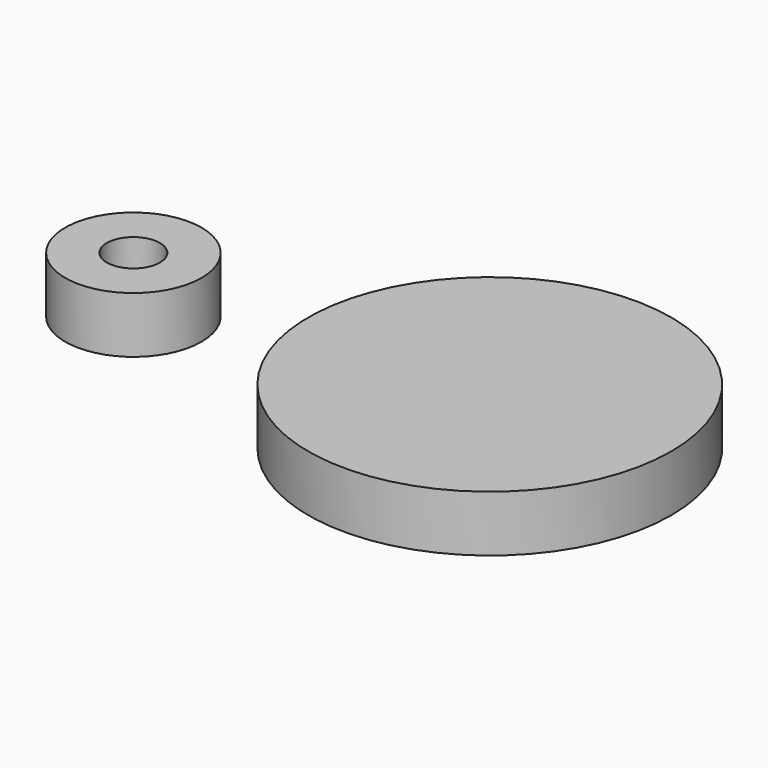
from build123d import *

# Parameters (mm, degrees)
F0_R     = 3.85
F0_R_2   = 1.5
F1_DEPTH = 3.175
F0_R_3   = 10.25


# Not quite as in the source:
# - a length typed as a fraction of an inch, garbled in the dataset ("3 / 203.2 mm" for 3/8 in), is restored


with BuildPart() as f1:
    # F0 (on Top) → F1 (new body)
    with BuildSketch(Plane.XY):
        Circle(F0_R)
        Circle(F0_R_2, mode=Mode.SUBTRACT)
    extrude(amount=F1_DEPTH)


with BuildPart() as f1b:
    # F0 (on Top) → F1, piece 2 (new body)
    with BuildSketch(Plane.XY):
        with Locations((20.1293285936, 0)):
            Circle(F0_R_3)
    extrude(amount=F1_DEPTH)


solid = Compound([f1.part, f1b.part])
